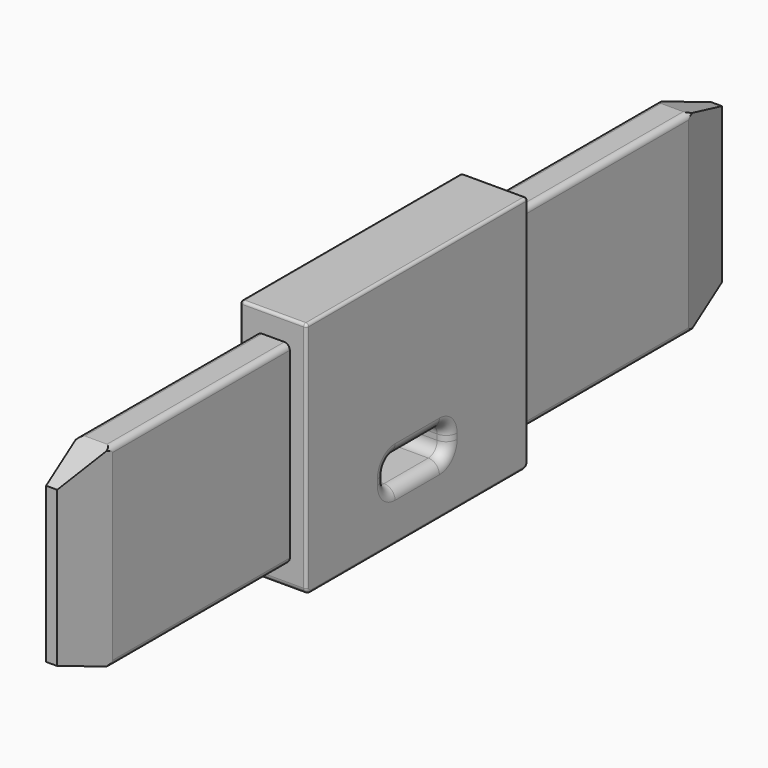
from build123d import *

# Parameters (mm, degrees)
F0_W          = 75
F0_H          = 35
F1_DEPTH      = 3
F4_W          = 10.7173770666
F4_H          = 34.9826700985
F5_DEPTH      = 25
F7_W          = 6
F7_H          = 35
F7_W_2        = 2
F7_H_2        = 28
F8_DEPTH      = 10
F9_DEPTH      = 10
F9_FACE_W     = 6
F9_FACE_H     = 35
F11_W         = 2
F11_H         = 28
F14_DEPTH     = 6
F16_DEPTH     = 25
F17_R         = 2
F18_R         = 0.5
F20_T1_DEPTH  = 12
F20_T4_ANGLE  = 90
F20_T6_ANGLE  = 90
F20_T8_ANGLE  = 90
F20_T10_ANGLE = 90
F21_R         = 1


# Not quite as in the source:
# - a fillet or chamfer that OpenCascade refuses, or shapes differently, is made with other operations: its cross-section is extruded or revolved along the edge and cut away or added
# - a feature of the source that left no trace in its solid (it failed there, or was rolled back) is left out
# - a feature names something its author has since deleted; it is built from what else it names


with BuildPart() as f1:
    # F0 (on Right) → F1 (new body, symmetric)
    with BuildSketch(Plane.YZ):
        with Locations((37.5, 0)):
            Rectangle(F0_W, F0_H)
    extrude(amount=F1_DEPTH, both=True)

    # F4 (on offset) → F5 (cut)
    with BuildSketch(Plane.XZ.offset(-10)):
        Rectangle(F4_W, F4_H)
    extrude(amount=F5_DEPTH, mode=Mode.SUBTRACT)

    # F7 (on face) → F8 (cut)
    with BuildSketch(Plane(origin=(0, 75, 0), x_dir=(-1, 0, 0), z_dir=(0, 1, 0))):
        Rectangle(F7_W, F7_H)
        Rectangle(F7_W_2, F7_H_2, mode=Mode.SUBTRACT)
    extrude(amount=F8_DEPTH, mode=Mode.SUBTRACT)

    # F9 (cut): a face of the model
    f9_faces = [f1.faces().sort_by_distance(p)[0] for p in [
        (0, 75, 0),
    ]]
    extrude(f9_faces, amount=-F9_DEPTH, mode=Mode.SUBTRACT)

    # F9_face (on face) → F12 section 0
    with BuildSketch(Plane(origin=(0, 65, 0), x_dir=(-1, 0, 0), z_dir=(0, 1, 0))):
        Rectangle(F9_FACE_W, F9_FACE_H)
    # F11 (on offset) → F12 section 1
    with BuildSketch(Plane(origin=(0, 75, 0), x_dir=(-1, 0, 0), z_dir=(0, 1, 0))):
        Rectangle(F11_W, F11_H)
    loft()

    # F13 (on Right) → F14 (join, symmetric)
    with BuildSketch(Plane.YZ):
        Polygon((25, 21.5), (0, 21.5), (-25, 21.5), (-25, 0), (-25, -21.5), (0, -21.5), (25, -21.5), (25, 0), align=None)
    extrude(amount=F14_DEPTH, both=True)

    # F15 (on face) → F16 (cut)
    with BuildSketch(Plane(origin=(-6, 0, 0), x_dir=(0, -1, 0), z_dir=(-1, 0, 0))):
        with BuildLine():
            Line((-5, -12.5), (5, -12.5))
            ThreePointArc((5, -12.5), (6.4142135624, -11.9142135624), (7, -10.5))
            Line((7, -10.5), (7, -9.5))
            ThreePointArc((7, -9.5), (6.4142135624, -8.0857864376), (5, -7.5))
            Line((5, -7.5), (-5, -7.5))
            ThreePointArc((-5, -7.5), (-6.4142135624, -8.0857864376), (-7, -9.5))
            Line((-7, -9.5), (-7, -10.5))
            ThreePointArc((-7, -10.5), (-6.4142135624, -11.9142135624), (-5, -12.5))
        make_face()
    extrude(amount=-F16_DEPTH, mode=Mode.SUBTRACT)

    # F17
    f17_edges = [f1.edges().sort_by_distance(p)[0] for p in [
        (6, 0, -7.5),
        (6, -6.414214, -8.085786),
        (6, -7, -10),
        (6, -6.414214, -11.914214),
        (6, 0, -12.5),
        (6, 6.414214, -8.085786),
        (6, 7, -10),
        (6, 6.414214, -11.914214),
        (-6, 0, -7.5),
        (-6, -6.414214, -8.085786),
        (-6, -7, -10),
        (-6, -6.414214, -11.914214),
        (-6, 0, -12.5),
        (-6, 6.414214, -11.914214),
        (-6, 7, -10),
        (-6, 6.414214, -8.085786),
    ]]
    fillet(f17_edges, radius=F17_R)

    # F18
    f18_edges = [f1.edges().sort_by_distance(p)[0] for p in [
        (-6, 0, 21.5),
        (0, -25, 21.5),
        (6, 0, 21.5),
        (0, 25, 21.5),
        (6, 0, -5.5),
        (6, 7.828427, -6.671573),
        (6, -7.828427, -6.671573),
        (6, 9, -10),
        (6, -9, -10),
        (6, 7.828427, -13.328427),
        (6, -7.828427, -13.328427),
        (6, 0, -14.5),
        (6, -25, 0),
        (6, 25, 0),
        (6, 0, -21.5),
        (-6, 0, -5.5),
        (-6, -7.828427, -6.671573),
        (-6, 7.828427, -6.671573),
        (-6, -9, -10),
        (-6, 9, -10),
        (-6, -7.828427, -13.328427),
        (-6, 7.828427, -13.328427),
        (-6, 0, -14.5),
        (-6, 25, 0),
        (-6, -25, 0),
        (-6, 0, -21.5),
    ]]
    fillet(f18_edges, radius=F18_R)

    # F19: F1 across plane


with BuildPart() as f1_1:
    add(f1.part)
    add(f1.part.mirror(Plane.XZ))

    # F20: fillet of radius 1 on 2 edges, made by hand

    # F20_s2 → F20_t1 (cut)
    with BuildSketch(Plane.YZ.offset(-6)):
        with BuildLine():
            ThreePointArc((25, -20.5), (24.7071067812, -21.2071067812), (24, -21.5))
            Line((24, -21.5), (25, -21.5))
            Line((25, -21.5), (25, -20.5))
        make_face()
        with BuildLine():
            ThreePointArc((-25, -20.5), (-24.7071067812, -21.2071067812), (-24, -21.5))
            Line((-24, -21.5), (-25, -21.5))
            Line((-25, -21.5), (-25, -20.5))
        make_face()
    extrude(amount=F20_T1_DEPTH, mode=Mode.SUBTRACT)

    # F20_s3 → F20_t4 (revolve, cut)
    with BuildSketch(Plane.XZ.offset(24)):
        with BuildLine():
            ThreePointArc((-6, -21), (-5.8535533906, -21.3535533906), (-5.5, -21.5))
            Line((-5.5, -21.5), (-6, -21.5))
            Line((-6, -21.5), (-6, -21))
        make_face()
    revolve(axis=Axis((-6, -24, -20.5), (-1, 0, 0)), revolution_arc=F20_T4_ANGLE, mode=Mode.SUBTRACT)

    # F20_s5 → F20_t6 (revolve, cut)
    with BuildSketch(Plane.XY.offset(-20.5)):
        with BuildLine():
            ThreePointArc((6, -24.5), (5.8535533906, -24.8535533906), (5.5, -25))
            Line((5.5, -25), (6, -25))
            Line((6, -25), (6, -24.5))
        make_face()
    revolve(axis=Axis((6, -24, -20.5), (1, 0, 0)), revolution_arc=F20_T6_ANGLE, mode=Mode.SUBTRACT)

    # F20_s7 → F20_t8 (revolve, cut)
    with BuildSketch(Plane.XZ.offset(-24)):
        with BuildLine():
            ThreePointArc((6, -21), (5.8535533906, -21.3535533906), (5.5, -21.5))
            Line((5.5, -21.5), (6, -21.5))
            Line((6, -21.5), (6, -21))
        make_face()
    revolve(axis=Axis((6, 24, -20.5), (1, 0, 0)), revolution_arc=F20_T8_ANGLE, mode=Mode.SUBTRACT)

    # F20_s9 → F20_t10 (revolve, cut)
    with BuildSketch(Plane.XY.offset(-20.5)):
        with BuildLine():
            ThreePointArc((-6, 24.5), (-5.8535533906, 24.8535533906), (-5.5, 25))
            Line((-5.5, 25), (-6, 25))
            Line((-6, 25), (-6, 24.5))
        make_face()
    revolve(axis=Axis((-6, 24, -20.5), (-1, 0, 0)), revolution_arc=F20_T10_ANGLE, mode=Mode.SUBTRACT)

    # F21
    f21_edges = [f1_1.edges().sort_by_distance(p)[0] for p in [
        (3, 45, -17.5),
        (3, 45, 17.5),
        (-3, 45, 17.5),
        (-3, 45, -17.5),
        (-3, -45, 17.5),
        (-3, -45, -17.5),
        (3, -45, -17.5),
        (3, -45, 17.5),
    ]]
    fillet(f21_edges, radius=F21_R)


solid = f1_1.part
